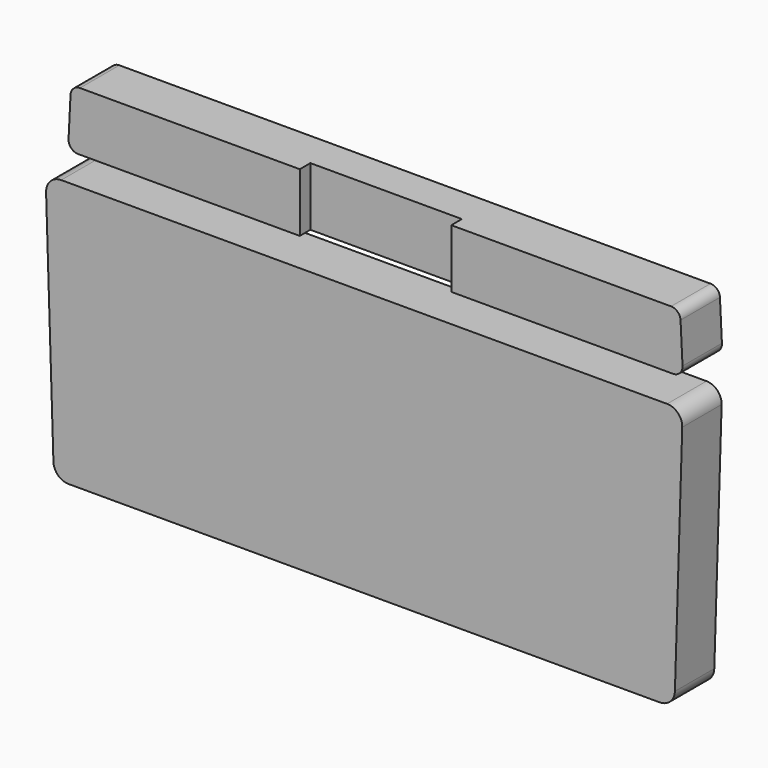
from build123d import *

# Parameters (mm, degrees)
F2_DEPTH  = 26
F4_DEPTH  = 26
F5_R      = 5
F6_W      = 80
F6_H      = 36
F7_DEPTH  = 7
F8_R      = 8
F11_W     = 342.5
F11_H     = 418.889449735
F12_DEPTH = 26.001


with BuildPart() as f2:
    # F1 (on Front) → F2 (new body)
    with BuildSketch(Plane.XZ):
        Polygon((-157.8051775685, -151), (-100.5, -151), (100.5, -151), (152.5, -151), (169.8110355137, -151), (174.1860355137, -11), (-162.1801775685, -11), (-159.6801775685, -91), align=None)
    extrude(amount=F2_DEPTH)

    # F8
    f8_edges = [f2.edges().sort_by_distance(p)[0] for p in [
        (169.811036, -13, -151),
        (-162.180178, -13, -11),
        (174.186036, -13, -11),
        (-157.805178, -13, -151),
    ]]
    fillet(f8_edges, radius=F8_R)


with BuildPart() as f4:
    # F3 (on Front) → F4 (new body)
    with BuildSketch(Plane.XZ):
        Polygon((-162.3312617041, 4), (162.3312617041, 4), (160.7812617041, 35), (-160.7812617041, 35), align=None)
    extrude(amount=F4_DEPTH)

    # F5
    f5_edges = [f4.edges().sort_by_distance(p)[0] for p in [
        (-160.781262, -13, 35),
        (-162.331262, -13, 4),
        (160.781262, -13, 35),
        (162.331262, -13, 4),
    ]]
    fillet(f5_edges, radius=F5_R)

    # F6 (on face) → F7 (cut)
    with BuildSketch(Plane.XZ.offset(26)):
        with Locations((0, 17)):
            Rectangle(F6_W, F6_H)
    extrude(amount=-F7_DEPTH, mode=Mode.SUBTRACT)


with BuildPart() as f10_1:
    # F10: instance of F4
    add(f4.part.mirror(Plane.YZ.offset(-165)))


with BuildPart() as f10_2:
    # F10: instance of F2
    add(f2.part.mirror(Plane.YZ.offset(-165)))


with BuildPart() as f12_tool:
    # F11 (on Front) → F12 (new body, through all)
    with BuildSketch(Plane.XZ):
        with Locations((6.25, 0)):
            Rectangle(F11_W, F11_H)
    extrude(amount=F12_DEPTH)


with BuildPart() as f2_1:
    add(f2.part)

    # F12: cut by f12_tool
    add(f12_tool.part, mode=Mode.SUBTRACT)


with BuildPart() as f4_1:
    add(f4.part)

    # F12: cut by f12_tool
    add(f12_tool.part, mode=Mode.SUBTRACT)


solid = Compound([f10_1.part, f10_2.part])
